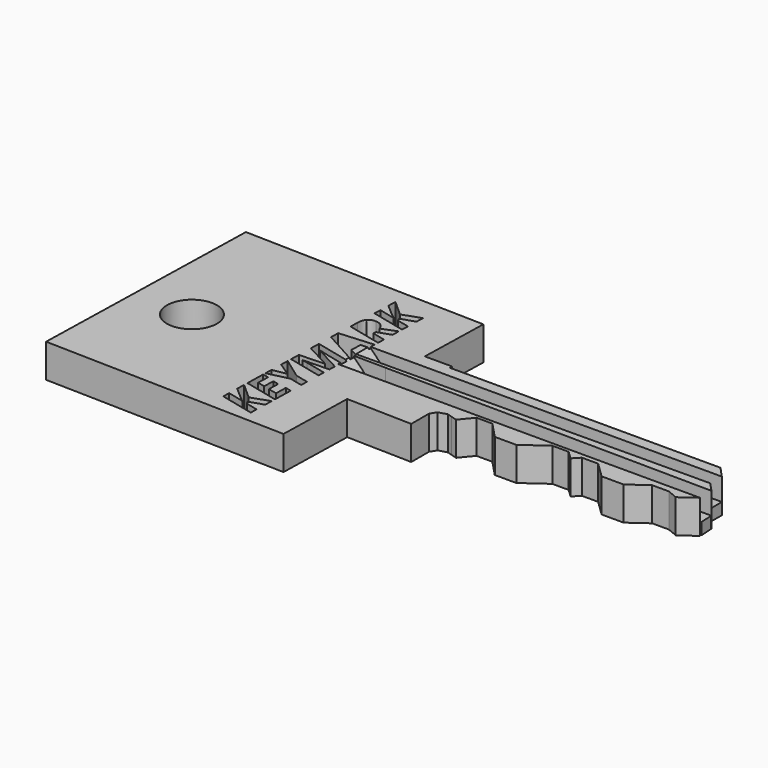
from build123d import *

# Parameters (mm, degrees)
F2_DEPTH     = 3.05
F3_DEPTH     = 1.06
F4_T4_DEPTH  = 9.2120308166
F4_T11_DEPTH = 9.2120308166
F4_T18_DEPTH = 9.2120308166
F4_T25_DEPTH = 9.2120308166
F4_T31_DEPTH = 9.2120308166
F5_T4_DEPTH  = 9.379453283
F5_T10_DEPTH = 9.379453283
F5_T16_DEPTH = 9.379453283
F5_T23_DEPTH = 9.379453283
F5_T30_DEPTH = 9.379453283
F6_R         = 2.2723720955
F7_DEPTH     = 8.9


# Not quite as in the source:
# - a fillet or chamfer that OpenCascade refuses, or shapes differently, is made with other operations: its cross-section is extruded or revolved along the edge and cut away or added


with BuildPart() as f2:
    # F0 (on Top) → F2 (new body)
    with BuildSketch(Plane.XY):
        Polygon((-58.7120377364, -11.5877003633), (-36.7188685864, -12.1358889587), (-36.5441002128, -5.1242319602), (-30.6113659254, -5.2721077508), (-30.6113659254, -3.2476347405), (-30.2592162043, -2.7069519274), (-29.4912289828, -2.4910855573), (-29.0750022978, -2.6250882074), (-28.5319797695, -2.7782688849), (-27.5932475924, -1.6439672327), (-26.1460356414, -1.6439672327), (-24.7379373759, -3.1302934512), (-22.7822437882, -3.1302934512), (-20.7092110068, -1.6439672327), (-19.2228853703, -1.6439672327), (-18.4797216207, -2.3480164818), (-17.9277884974, -1.7654198952), (-16.4458025247, -1.7654198952), (-15.0377042592, -3.1302934512), (-13.0428988487, -3.1302934512), (-11.3983151047, -1.9511572798), (-9.8746763542, -1.9511572798), (-8.9359441772, -2.3480164818), (-7.5324275531, -1.3417209832), (-37.4155603349, -1.3417209832), (-37.4155603349, 0.322683336), (-7.565138326, 0), (-8.3618185489, 0.8518604273), (-37.3642847361, 0.6698103581), (-37.3642847361, 2.1667922108), (-8.3618185489, 2.1667922108), (-9.2879692093, 3.1670355238), (-33.8603667915, 3.1670355238), (-36.3374370328, 3.1670355238), (-36.3310827873, 3.4219660304), (-36.170679991, 9.8572801914), (-58.1638491411, 10.4054687867), align=None)
        Polygon((-42.1491555744, -9.2971004325), (-40.5186647927, -8.7200768568), (-40.536536189, -9.4370721469), (-41.8025896769, -9.8528127458), (-41.6606462024, -10.1217427308), (-40.5600378359, -10.3799514782), (-40.5761508356, -11.026400401), (-43.6591267891, -10.2945604157), (-43.6429461588, -9.6453981711), (-42.1627202807, -10.0047005421), (-42.5891946256, -9.6594458184), (-43.6210338319, -8.7662819025), (-43.6019450841, -8.0004468197), align=None, mode=Mode.SUBTRACT)
        Polygon((-41.0064807081, -6.5060467358), (-40.4666737393, -6.6342107103), (-40.5098389944, -8.3659883597), (-43.5928149479, -7.6341483745), (-43.5495820621, -5.8996574032), (-43.013845076, -6.0277199317), (-43.0408973315, -7.1130486584), (-42.3640824945, -7.2724564364), (-42.3388731739, -6.2610657292), (-41.8031869108, -6.3911632491), (-41.8283793237, -7.4018756258), (-41.0335329636, -7.5913754624), align=None, mode=Mode.SUBTRACT)
        Polygon((-43.5269765212, -4.992729586), (-42.2652513941, -4.7506415833), (-43.5003976802, -3.926394112), (-43.482323392, -3.2012588565), (-41.6007235412, -4.5588283791), (-40.4219698871, -4.8407049895), (-40.4379814408, -5.4830839296), (-41.6167350949, -5.2012073192), (-43.5434614893, -5.6541017788), align=None, mode=Mode.SUBTRACT)
        with BuildLine():
            Line((-41.1310269034, -1.8901445654), (-41.1308071038, -1.8813262695))
            Line((-41.1308071038, -1.8813262695), (-43.4188689453, -0.6554846621))
            Line((-43.4188689453, -0.6554846621), (-43.3965170192, 0.2412681983))
            Line((-43.3965170192, 0.2412681983), (-40.3135579734, -0.4912501174))
            Line((-40.3135579734, -0.4912501174), (-40.3283521756, -1.0847892648))
            Line((-40.3283521756, -1.0847892648), (-41.7879217781, -0.7409343012))
            add(Edge.make_bspline(
                [(-41.7879217781, -0.7409343012), (-42.3081078868, -0.6152956402), (-42.7171154316, -0.4951431572)],
                knots=[0, 0, 0, 1, 1, 1], degree=2))
            Line((-42.7171154316, -0.4951431572), (-42.7173690465, -0.505318114))
            Line((-42.7173690465, -0.505318114), (-40.3454796348, -1.7719380148))
            Line((-40.3454796348, -1.7719380148), (-40.36032456, -2.3675121536))
            Line((-40.36032456, -2.3675121536), (-42.7655051535, -2.436524917))
            Line((-42.7655051535, -2.436524917), (-42.7657249531, -2.4453432129))
            add(Edge.make_bspline(
                [(-42.7657249531, -2.4453432129), (-42.5797589386, -2.4730560548), (-42.2779739229, -2.537932702)],
                knots=[0, 0, 0, 1, 1, 1], degree=2))
            add(Edge.make_bspline(
                [(-42.2779739229, -2.537932702), (-41.9761889071, -2.6028093493), (-40.3756428997, -2.9820795451)],
                knots=[0, 0, 0, 1, 1, 1], degree=2))
            Line((-40.3756428997, -2.9820795451), (-40.3901665793, -3.5647654052))
            Line((-40.3901665793, -3.5647654052), (-43.4731425328, -2.8329254199))
            Line((-43.4731425328, -2.8329254199), (-43.4517881587, -1.9761940563))
            Line((-43.4517881587, -1.9761940563), (-41.1310269034, -1.8901445654))
        make_face(mode=Mode.SUBTRACT)
        Polygon((-40.2520140922, 1.9778727358), (-40.9913057008, 1.9453934854), (-41.0162952218, 0.9428210742), (-40.2873511009, 0.5601620866), (-40.3042587606, -0.1181683676), (-43.3759788547, 1.5826487517), (-43.3562645235, 2.3735820613), (-40.2363237841, 2.6073633972), align=None, mode=Mode.SUBTRACT)
        with BuildLine():
            Line((-41.3874286513, 4.1618893856), (-41.3937183007, 3.9095504566))
            Line((-41.3937183007, 3.9095504566), (-40.2108946639, 3.6275724003))
            Line((-40.2108946639, 3.6275724003), (-40.2270076636, 2.9811234775))
            Line((-40.2270076636, 2.9811234775), (-43.3099836171, 3.7129634627))
            Line((-43.3099836171, 3.7129634627), (-43.2910132229, 4.4740502323))
            add(Edge.make_bspline(
                [(-43.2910132229, 4.4740502323), (-43.2784846471, 4.9766930988), (-43.0558075829, 5.2236384844)],
                knots=[0, 0, 0, 1, 1, 1], degree=2))
            add(Edge.make_bspline(
                [(-43.0558075829, 5.2236384844), (-42.8331305186, 5.4705838699), (-42.4159572893, 5.4601856592)],
                knots=[0, 0, 0, 1, 1, 1], degree=2))
            add(Edge.make_bspline(
                [(-42.4159572893, 5.4601856592), (-42.0808620449, 5.4518332753), (-41.8447814366, 5.2698127571)],
                knots=[0, 0, 0, 1, 1, 1], degree=2))
            add(Edge.make_bspline(
                [(-41.8447814366, 5.2698127571), (-41.6087008283, 5.0877922389), (-41.5002789281, 4.7538588598)],
                knots=[0, 0, 0, 1, 1, 1], degree=2))
            Line((-41.5002789281, 4.7538588598), (-40.1698428663, 5.274558743))
            Line((-40.1698428663, 5.274558743), (-40.187393017, 4.5704517316))
            Line((-40.187393017, 4.5704517316), (-41.3874286513, 4.1618893856))
        make_face(mode=Mode.SUBTRACT)
        Polygon((-41.7341232527, 7.3538772259), (-40.103632471, 7.9309008015), (-40.1215038673, 7.2139055115), (-41.3875573552, 6.7981649125), (-41.2456138807, 6.5292349275), (-40.1450055142, 6.2710261802), (-40.1611185139, 5.6245772574), (-43.2440944674, 6.3564172426), (-43.2279138371, 7.0055794872), (-41.747687959, 6.6462771162), (-42.1741623039, 6.99153184), (-43.2060015102, 7.8846957558), (-43.1869127624, 8.6505308386), align=None, mode=Mode.SUBTRACT)
        Polygon((-33.8603667915, 3.4219660304), (-36.3310827873, 3.4219660304), (-36.3374370328, 3.1670355238), (-33.8603667915, 3.1670355238), align=None)
    extrude(amount=F2_DEPTH)

    # F1 (on Top) → F3 (join)
    with BuildSketch(Plane.XY):
        Polygon((-38.6960990727, -1.2029025238), (-7.5144232251, -1.2029025238), (-7.5898682699, 0), (-38.6166758835, 0), align=None)
        Polygon((-38.6166758835, 0.7971409359), (-8.3092655987, 0.7971409359), (-8.3098765463, 2.1124139894), (-38.5213717818, 2.1124139894), align=None)
    extrude(amount=F3_DEPTH)

    # F4: chamfer of 3 on 1 edges, made by hand


with BuildPart() as f4_tool2:
    # F4_s3 → F4_t4 (new body)
    with BuildSketch(Plane.XZ.offset(7.0452386058)):
        with BuildLine():
            Line((-40.4491375499, 3.1348528137), (-37.2794319224, -0.0348528137))
            Line((-37.2794319224, -0.0348528137), (-37.2194319224, -0.0348528137))
            ThreePointArc((-37.2194319224, -0.0348528137), (-37.3042847361, 1.5075735931), (-37.3042847361, 3.05))
            Line((-37.3042847361, 3.05), (-37.3642847361, 3.11))
            ThreePointArc((-37.3642847361, 3.11), (-38.906711143, 3.11), (-40.4491375499, 3.1948528137))
            Line((-40.4491375499, 3.1948528137), (-40.4491375499, 3.1348528137))
        make_face()
    extrude(amount=-F4_T4_DEPTH)

    split(bisect_by=Plane.XZ.offset(-0.7971409359), keep=Keep.TOP)

    split(bisect_by=Plane.XY.offset(1.06), keep=Keep.TOP)

    split(bisect_by=Plane(origin=(-0.0056764184, 0.9043123893, 0), x_dir=(0, 0, 1), z_dir=(-0.0062769311, 0.9999802999, 0)), keep=Keep.TOP)


with BuildPart() as f2_1:
    add(f2.part)

    # F4_t1: cut F4_tool2
    add(f4_tool2.part, mode=Mode.SUBTRACT)


with BuildPart() as f4_tool9:
    # F4_s10 → F4_t11 (new body)
    with BuildSketch(Plane.XZ.offset(7.0452386058)):
        with BuildLine():
            Line((-40.4491375499, 3.1348528137), (-37.2794319224, -0.0348528137))
            Line((-37.2794319224, -0.0348528137), (-37.2194319224, -0.0348528137))
            ThreePointArc((-37.2194319224, -0.0348528137), (-37.3042847361, 1.5075735931), (-37.3042847361, 3.05))
            Line((-37.3042847361, 3.05), (-37.3642847361, 3.11))
            ThreePointArc((-37.3642847361, 3.11), (-38.906711143, 3.11), (-40.4491375499, 3.1948528137))
            Line((-40.4491375499, 3.1948528137), (-40.4491375499, 3.1348528137))
        make_face()
    extrude(amount=-F4_T11_DEPTH)

    split(bisect_by=Plane.XZ.offset(-0.7971409359), keep=Keep.TOP)

    split(bisect_by=Plane.XY.offset(1.06), keep=Keep.BOTTOM)

    split(bisect_by=Plane(origin=(-0.0056764184, 0.9043123893, 0), x_dir=(0, 0, 1), z_dir=(-0.0062769311, 0.9999802999, 0)), keep=Keep.TOP)


with BuildPart() as f2_2:
    add(f2_1.part)

    # F4_t8: cut F4_tool9
    add(f4_tool9.part, mode=Mode.SUBTRACT)


with BuildPart() as f4_tool16:
    # F4_s17 → F4_t18 (new body)
    with BuildSketch(Plane.XZ.offset(7.0452386058)):
        with BuildLine():
            Line((-40.4491375499, 3.1348528137), (-37.2794319224, -0.0348528137))
            Line((-37.2794319224, -0.0348528137), (-37.2194319224, -0.0348528137))
            ThreePointArc((-37.2194319224, -0.0348528137), (-37.3042847361, 1.5075735931), (-37.3042847361, 3.05))
            Line((-37.3042847361, 3.05), (-37.3642847361, 3.11))
            ThreePointArc((-37.3642847361, 3.11), (-38.906711143, 3.11), (-40.4491375499, 3.1948528137))
            Line((-40.4491375499, 3.1948528137), (-40.4491375499, 3.1348528137))
        make_face()
    extrude(amount=-F4_T18_DEPTH)

    split(bisect_by=Plane.XZ.offset(-0.7971409359), keep=Keep.BOTTOM)

    split(bisect_by=Plane.XY.offset(1.06), keep=Keep.TOP)

    split(bisect_by=Plane.XZ.offset(-2.1124139894), keep=Keep.TOP)


with BuildPart() as f2_3:
    add(f2_2.part)

    # F4_t15: cut F4_tool16
    add(f4_tool16.part, mode=Mode.SUBTRACT)


with BuildPart() as f4_tool23:
    # F4_s24 → F4_t25 (new body)
    with BuildSketch(Plane.XZ.offset(7.0452386058)):
        with BuildLine():
            Line((-40.4491375499, 3.1348528137), (-37.2794319224, -0.0348528137))
            Line((-37.2794319224, -0.0348528137), (-37.2194319224, -0.0348528137))
            ThreePointArc((-37.2194319224, -0.0348528137), (-37.3042847361, 1.5075735931), (-37.3042847361, 3.05))
            Line((-37.3042847361, 3.05), (-37.3642847361, 3.11))
            ThreePointArc((-37.3642847361, 3.11), (-38.906711143, 3.11), (-40.4491375499, 3.1948528137))
            Line((-40.4491375499, 3.1948528137), (-40.4491375499, 3.1348528137))
        make_face()
    extrude(amount=-F4_T25_DEPTH)

    split(bisect_by=Plane.XY.offset(1.06), keep=Keep.TOP)

    split(bisect_by=Plane.XZ.offset(-2.1124139894), keep=Keep.BOTTOM)


with BuildPart() as f2_4:
    add(f2_3.part)

    # F4_t22: cut F4_tool23
    add(f4_tool23.part, mode=Mode.SUBTRACT)


with BuildPart() as f4_tool29:
    # F4_s30 → F4_t31 (new body)
    with BuildSketch(Plane.XZ.offset(7.0452386058)):
        with BuildLine():
            Line((-40.4491375499, 3.1348528137), (-37.2794319224, -0.0348528137))
            Line((-37.2794319224, -0.0348528137), (-37.2194319224, -0.0348528137))
            ThreePointArc((-37.2194319224, -0.0348528137), (-37.3042847361, 1.5075735931), (-37.3042847361, 3.05))
            Line((-37.3042847361, 3.05), (-37.3642847361, 3.11))
            ThreePointArc((-37.3642847361, 3.11), (-38.906711143, 3.11), (-40.4491375499, 3.1948528137))
            Line((-40.4491375499, 3.1948528137), (-40.4491375499, 3.1348528137))
        make_face()
    extrude(amount=-F4_T31_DEPTH)

    split(bisect_by=Plane.XY.offset(1.06), keep=Keep.BOTTOM)

    split(bisect_by=Plane.XZ.offset(-2.1124139894), keep=Keep.BOTTOM)


with BuildPart() as f2_5:
    add(f2_4.part)

    # F4_t28: cut F4_tool29
    add(f4_tool29.part, mode=Mode.SUBTRACT)

    # F5: chamfer of 3 on 1 edges, made by hand


with BuildPart() as f5_tool2:
    # F5_s3 → F5_t4 (new body)
    with BuildSketch(Plane.XZ.offset(1.3417209832)):
        Polygon((-40.4155603349, 3.05), (-37.4155603349, 0.05), (-37.4155603349, 3.05), align=None)
    extrude(amount=-F5_T4_DEPTH)

    split(bisect_by=Plane.XZ.offset(1.2029025238), keep=Keep.TOP)

    split(bisect_by=Plane.XY.offset(1.06), keep=Keep.TOP)


with BuildPart() as f2_6:
    add(f2_5.part)

    # F5_t1: cut F5_tool2
    add(f5_tool2.part, mode=Mode.SUBTRACT)


with BuildPart() as f5_tool8:
    # F5_s9 → F5_t10 (new body)
    with BuildSketch(Plane.XZ.offset(1.3417209832)):
        Polygon((-40.4155603349, 3.05), (-37.4155603349, 0.05), (-37.4155603349, 3.05), align=None)
    extrude(amount=-F5_T10_DEPTH)

    split(bisect_by=Plane.XZ.offset(1.2029025238), keep=Keep.TOP)

    split(bisect_by=Plane.XY.offset(1.06), keep=Keep.BOTTOM)


with BuildPart() as f2_7:
    add(f2_6.part)

    # F5_t7: cut F5_tool8
    add(f5_tool8.part, mode=Mode.SUBTRACT)


with BuildPart() as f5_tool14:
    # F5_s15 → F5_t16 (new body)
    with BuildSketch(Plane.XZ.offset(1.3417209832)):
        Polygon((-40.4155603349, 3.05), (-37.4155603349, 0.05), (-37.4155603349, 3.05), align=None)
    extrude(amount=-F5_T16_DEPTH)

    split(bisect_by=Plane.XZ.offset(1.2029025238), keep=Keep.BOTTOM)

    split(bisect_by=Plane.XY.offset(1.06), keep=Keep.TOP)

    split(bisect_by=Plane.XZ, keep=Keep.TOP)


with BuildPart() as f2_8:
    add(f2_7.part)

    # F5_t13: cut F5_tool14
    add(f5_tool14.part, mode=Mode.SUBTRACT)


with BuildPart() as f5_tool21:
    # F5_s22 → F5_t23 (new body)
    with BuildSketch(Plane.XZ.offset(1.3417209832)):
        Polygon((-40.4155603349, 3.05), (-37.4155603349, 0.05), (-37.4155603349, 3.05), align=None)
    extrude(amount=-F5_T23_DEPTH)

    split(bisect_by=Plane(origin=(-0.0008839308, -0.0817696595, 0), x_dir=(0, 0, 1), z_dir=(-0.0108093776, -0.999941577, 0)), keep=Keep.TOP)

    split(bisect_by=Plane.XY.offset(1.06), keep=Keep.TOP)

    split(bisect_by=Plane.XZ, keep=Keep.BOTTOM)


with BuildPart() as f2_9:
    add(f2_8.part)

    # F5_t20: cut F5_tool21
    add(f5_tool21.part, mode=Mode.SUBTRACT)


with BuildPart() as f5_tool28:
    # F5_s29 → F5_t30 (new body)
    with BuildSketch(Plane.XZ.offset(1.3417209832)):
        Polygon((-40.4155603349, 3.05), (-37.4155603349, 0.05), (-37.4155603349, 3.05), align=None)
    extrude(amount=-F5_T30_DEPTH)

    split(bisect_by=Plane(origin=(-0.0008839308, -0.0817696595, 0), x_dir=(0, 0, 1), z_dir=(-0.0108093776, -0.999941577, 0)), keep=Keep.TOP)

    split(bisect_by=Plane.XY.offset(1.06), keep=Keep.BOTTOM)

    split(bisect_by=Plane.XZ, keep=Keep.BOTTOM)


with BuildPart() as f2_10:
    add(f2_9.part)

    # F5_t27: cut F5_tool28
    add(f5_tool28.part, mode=Mode.SUBTRACT)

    # F6 (on Top) → F7 (cut)
    with BuildSketch(Plane.XY):
        with Locations((-53.2489940524, -1.8617680762)):
            Circle(F6_R)
    extrude(amount=F7_DEPTH, mode=Mode.SUBTRACT)


solid = f2_10.part
